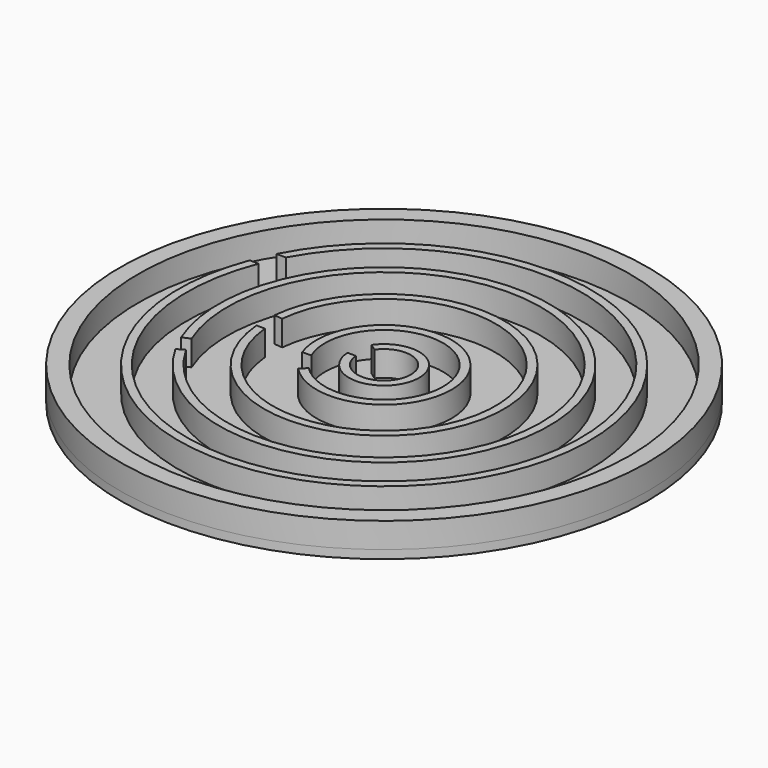
from build123d import *

# Parameters (mm, degrees)
F1_DEPTH = 6
F0_R     = 62.6558654543
F0_R_2   = 58.3558654543
F2_R     = 62.6558654543
F3_DEPTH = 2


with BuildPart() as f1:
    # F0 (on Top) → F1 (new body)
    with BuildSketch(Plane.XY):
        with BuildLine():
            Line((-43.5062726708, 17.1923115849), (-45.6499275725, 17.1923115849))
            ThreePointArc((-45.6499275725, 17.1923115849), (44.5938282764, -19.7707345503), (-43.392231874, 22.2846511751))
            Line((-43.392231874, 22.2846511751), (-41.1310790199, 22.2846511751))
            ThreePointArc((-41.1310790199, 22.2846511751), (42.3952038081, -19.7741759224), (-43.5062726708, 17.1923115849))
        make_face()
    extrude(amount=F1_DEPTH)


with BuildPart() as f1b:
    # F0 (on Top) → F1, piece 2 (new body)
    with BuildSketch(Plane.XY):
        Circle(F0_R)
        Circle(F0_R_2, mode=Mode.SUBTRACT)
    extrude(amount=F1_DEPTH)


with BuildPart() as f1c:
    # F0 (on Top) → F1, piece 3 (new body)
    with BuildSketch(Plane.XY):
        with BuildLine():
            Line((-32.4305662193, -18.2259800495), (-34.1740896291, -19.2058403045))
            ThreePointArc((-34.1740896291, -19.2058403045), (35.2911157623, 17.0666297797), (-36.2743942596, -14.862739481))
            Line((-36.2743942596, -14.862739481), (-34.4237156824, -14.104459319))
            ThreePointArc((-34.4237156824, -14.104459319), (33.4906029422, 16.1959096267), (-32.4305662193, -18.2259800495))
        make_face()
    extrude(amount=F1_DEPTH)


with BuildPart() as f1d:
    # F0 (on Top) → F1, piece 4 (new body)
    with BuildSketch(Plane.XY):
        with BuildLine():
            Line((-26.3380359585, -2.4378048256), (-28.3459802776, -2.4378048256))
            ThreePointArc((-28.3459802776, -2.4378048256), (28.4498566189, -0.2077224752), (-28.3073615488, 2.851450931))
            Line((-28.3073615488, 2.851450931), (-26.317431868, 2.6510017711))
            ThreePointArc((-26.317431868, 2.6510017711), (26.4503981284, -0.1070951284), (-26.3380359585, -2.4378048256))
        make_face()
    extrude(amount=F1_DEPTH)


with BuildPart() as f1e:
    # F0 (on Top) → F1, piece 5 (new body)
    with BuildSketch(Plane.XY):
        with BuildLine():
            Line((-10.069114881, -9.7412249533), (-11.5065388559, -11.131840758))
            ThreePointArc((-11.5065388559, -11.131840758), (13.5703952835, 8.4948623858), (-15.0405875779, -5.4862592369))
            Line((-15.0405875779, -5.4862592369), (-12.8910627049, -5.4862592369))
            ThreePointArc((-12.8910627049, -5.4862592369), (11.6755566037, 7.7433788537), (-10.069114881, -9.7412249533))
        make_face()
    extrude(amount=F1_DEPTH)


with BuildPart() as f1f:
    # F0 (on Top) → F1, piece 6 (new body)
    with BuildSketch(Plane.XY):
        with BuildLine():
            ThreePointArc((-5.1794242353, 3.646916388), (6.1038145867, -1.6940726198), (-6.3181195634, -0.4558505607))
            Line((-6.3181195634, -0.4558505607), (-8.3220673289, -0.4558505607))
            ThreePointArc((-8.3220673289, -0.4558505607), (8.0113822453, -2.2983382867), (-6.8147194565, 4.7983542063))
            Line((-6.8147194565, 4.7983542063), (-5.1794242353, 3.646916388))
        make_face()
    extrude(amount=F1_DEPTH)


with BuildPart() as f3:
    # F2 (on Top) → F3 (new body)
    with BuildSketch(Plane.XY):
        Circle(F2_R)
    extrude(amount=-F3_DEPTH)


solid = Compound([f1.part, f1b.part, f1c.part, f1d.part, f1e.part, f1f.part, f3.part])
